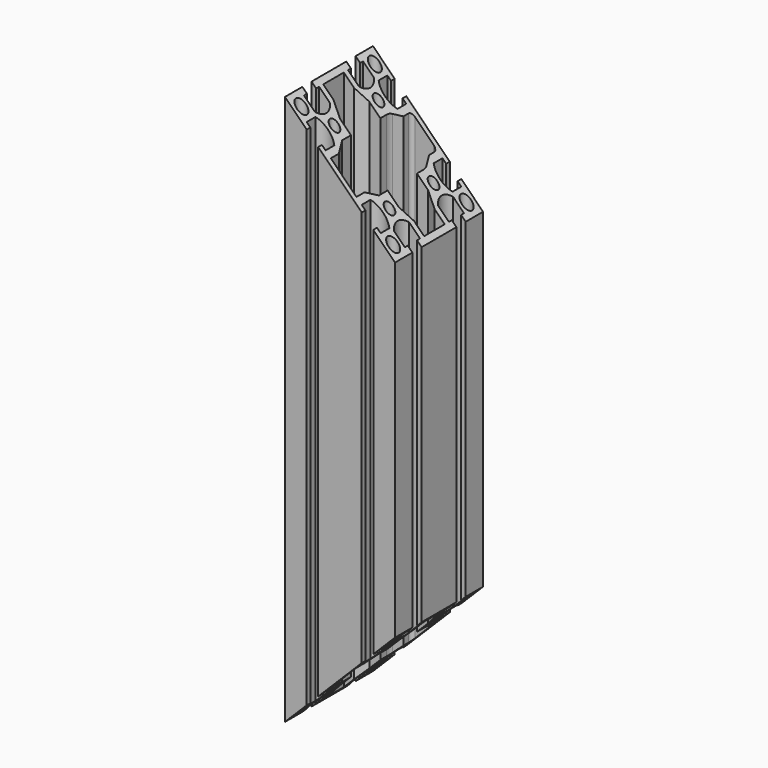
from build123d import *

# Parameters (mm, degrees)
F0_R          = 3
F0_R_2        = 2.5
F1_DEPTH      = 300
F2_R          = 2
F3_R          = 7
F6_DEPTH      = 30
F6_DEPTH_BACK = 30


# Not quite as in the source:
# - a feature names something its author has since deleted; it is built from what else it names


with BuildPart() as f1:
    # F0 (on Top) → F1 (new body)
    with BuildSketch(Plane.XY):
        with BuildLine():
            Line((18.15, -30), (30, -30))
            Line((30, -30), (30, -18.15))
            Line((30, -18.15), (27.5, -18.15))
            Line((27.5, -18.15), (27.5, -20.15))
            Line((27.5, -20.15), (21.5477069044, -20.15))
            ThreePointArc((21.5477069044, -20.15), (19.5, -15), (21.5477069044, -9.85))
            Line((21.5477069044, -9.85), (27.5, -9.85))
            Line((27.5, -9.85), (27.5, -11.85))
            Line((27.5, -11.85), (30, -11.85))
            Line((30, -11.85), (30, 11.85))
            Line((30, 11.85), (27.5, 11.85))
            Line((27.5, 11.85), (27.5, 9.85))
            Line((27.5, 9.85), (21.5477069044, 9.85))
            ThreePointArc((21.5477069044, 9.85), (19.5, 15), (21.5477069044, 20.15))
            Line((21.5477069044, 20.15), (27.5, 20.15))
            Line((27.5, 20.15), (27.5, 18.15))
            Line((27.5, 18.15), (30, 18.15))
            Line((30, 18.15), (30, 30))
            Line((30, 30), (18.15, 30))
            Line((18.15, 30), (18.15, 27.5))
            Line((18.15, 27.5), (20.15, 27.5))
            Line((20.15, 27.5), (20.15, 21.5477069044))
            ThreePointArc((20.15, 21.5477069044), (15, 19.5), (9.85, 21.5477069044))
            Line((9.85, 21.5477069044), (9.85, 27.5))
            Line((9.85, 27.5), (11.85, 27.5))
            Line((11.85, 27.5), (11.85, 30))
            Line((11.85, 30), (-11.85, 30))
            Line((-11.85, 30), (-11.85, 27.5))
            Line((-11.85, 27.5), (-9.85, 27.5))
            Line((-9.85, 27.5), (-9.85, 21.5477069044))
            ThreePointArc((-9.85, 21.5477069044), (-15, 19.5), (-20.15, 21.5477069044))
            Line((-20.15, 21.5477069044), (-20.15, 27.5))
            Line((-20.15, 27.5), (-18.15, 27.5))
            Line((-18.15, 27.5), (-18.15, 30))
            Line((-18.15, 30), (-30, 30))
            Line((-30, 30), (-30, 18.15))
            Line((-30, 18.15), (-27.5, 18.15))
            Line((-27.5, 18.15), (-27.5, 20.15))
            Line((-27.5, 20.15), (-21.5477069044, 20.15))
            ThreePointArc((-21.5477069044, 20.15), (-19.5, 15), (-21.5477069044, 9.85))
            Line((-21.5477069044, 9.85), (-27.5, 9.85))
            Line((-27.5, 9.85), (-27.5, 11.85))
            Line((-27.5, 11.85), (-30, 11.85))
            Line((-30, 11.85), (-30, -11.85))
            Line((-30, -11.85), (-27.5, -11.85))
            Line((-27.5, -11.85), (-27.5, -9.85))
            Line((-27.5, -9.85), (-21.5477069044, -9.85))
            ThreePointArc((-21.5477069044, -9.85), (-19.5, -15), (-21.5477069044, -20.15))
            Line((-21.5477069044, -20.15), (-27.5, -20.15))
            Line((-27.5, -20.15), (-27.5, -18.15))
            Line((-27.5, -18.15), (-30, -18.15))
            Line((-30, -18.15), (-30, -30))
            Line((-30, -30), (-18.15, -30))
            Line((-18.15, -30), (-18.15, -27.5))
            Line((-18.15, -27.5), (-20.15, -27.5))
            Line((-20.15, -27.5), (-20.15, -21.5477069044))
            ThreePointArc((-20.15, -21.5477069044), (-15, -19.5), (-9.85, -21.5477069044))
            Line((-9.85, -21.5477069044), (-9.85, -27.5))
            Line((-9.85, -27.5), (-11.85, -27.5))
            Line((-11.85, -27.5), (-11.85, -30))
            Line((-11.85, -30), (11.85, -30))
            Line((11.85, -30), (11.85, -27.5))
            Line((11.85, -27.5), (9.85, -27.5))
            Line((9.85, -27.5), (9.85, -21.5477069044))
            ThreePointArc((9.85, -21.5477069044), (15, -19.5), (20.15, -21.5477069044))
            Line((20.15, -21.5477069044), (20.15, -27.5))
            Line((20.15, -27.5), (18.15, -27.5))
            Line((18.15, -27.5), (18.15, -30))
        make_face()
        with Locations((-25, -25)):
            Circle(F0_R, mode=Mode.SUBTRACT)
        with Locations((-15, -15)):
            Circle(F0_R_2, mode=Mode.SUBTRACT)
        with Locations((25, -25)):
            Circle(F0_R, mode=Mode.SUBTRACT)
        with Locations((15, -15)):
            Circle(F0_R_2, mode=Mode.SUBTRACT)
        with Locations((-25, 25)):
            Circle(F0_R, mode=Mode.SUBTRACT)
        with Locations((-15, 15)):
            Circle(F0_R_2, mode=Mode.SUBTRACT)
        Polygon((-7, 22), (-7, 27.5), (0, 27.5), (7, 27.5), (7, 22), (10, 16), (10, 10), (16, 10), (22, 7), (27.5, 7), (27.5, 0), (27.5, -7), (22, -7), (16, -10), (10, -10), (10, -16), (7, -22), (7, -27.5), (0, -27.5), (-7, -27.5), (-7, -22), (-10, -16), (-10, -10), (-16, -10), (-22, -7), (-27.5, -7), (-27.5, 0), (-27.5, 7), (-22, 7), (-16, 10), (-10, 10), (-10, 16), align=None, mode=Mode.SUBTRACT)
        with Locations((15, 15)):
            Circle(F0_R_2, mode=Mode.SUBTRACT)
        with Locations((25, 25)):
            Circle(F0_R, mode=Mode.SUBTRACT)
    extrude(amount=F1_DEPTH)

    # F2
    f2_edges = [f1.edges().sort_by_distance(p)[0] for p in [
        (-7, 27.5, 150),
        (7, 27.5, 150),
    ]]
    fillet(f2_edges, radius=F2_R)

    # F3
    f3_edges = [f1.edges().sort_by_distance(p)[0] for p in [
        (-10, 16, 150),
        (10, 16, 150),
    ]]
    fillet(f3_edges, radius=F3_R)

    # F5 (on Front) → F6 (cut, two sides)
    with BuildSketch(Plane.XZ) as f6_sk:
        Polygon((144.6894081855, 37.2119464586), (75.9506773221, 105.9506773221), (-30, 0), (38.7387308634, -68.7387308634), align=None)
        Polygon((81.6358354247, 188.3641645753), (150.3745847274, 257.102913878), (38.7387493027, 368.7387493027), (-30, 300), align=None)
    extrude(amount=F6_DEPTH, mode=Mode.SUBTRACT)
    extrude(f6_sk.sketch, amount=-F6_DEPTH_BACK, mode=Mode.SUBTRACT)


solid = f1.part
